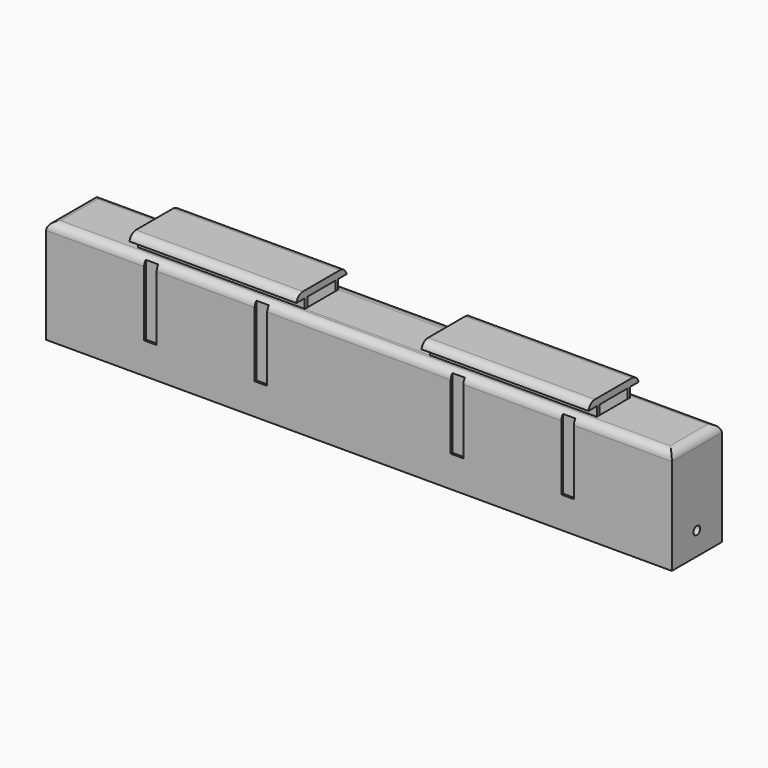
from build123d import *

# Parameters (mm, degrees)
F0_W           = 10.16
F0_H           = 2.54
F1_DEPTH       = 6.35
F2_DEPTH       = 0.635
F4_DEPTH       = 27.94
F6_R           = 0.254
F7_DEPTH       = 38.101
F8_T1_DEPTH    = 6.354829213
F8_T3_DEPTH    = 13.720829213
F10_DEPTH      = 9.652
F11_DEPTH      = 17.272
F12_W          = 2.5144716492
F12_H          = 3.5254987888
F13_DEPTH      = 3.81
F14_DEPTH      = 3.302
F16_DEPTH      = 10.16
F18_DEPTH      = 10.16
F20_DEPTH      = 10.16
F21_T1_DEPTH   = 12.6606557729
F23_DEPTH      = 10.16
F24_T1_DEPTH   = 12.6606557729
F24_2_T1_DEPTH = 8.0250460087
F24_2_T3_DEPTH = 8.0034146065
F24_2_T5_DEPTH = 8.0034146065
F24_2_T7_DEPTH = 8.0250460087
F25_W          = 7.62
F25_H          = 2.54
F26_DEPTH      = 4.5568268582
F27_W          = 7.62
F27_H          = 2.54
F28_DEPTH      = 4.5568268582
F0_W_2         = 0.762
F0_H_2         = 0.127
F29_DEPTH      = 1.905


# Not quite as in the source:
# - a fillet or chamfer that OpenCascade refuses, or shapes differently, is made with other operations: its cross-section is extruded or revolved along the edge and cut away or added


with BuildPart() as f1:
    # F0 (on Top) → F1 (new body)
    with BuildSketch(Plane.XY):
        Polygon((13.081, -1.905), (19.05, -1.905), (19.05, 1.905), (13.081, 1.905), (13.081, 1.778), (12.319, 1.778), (12.319, 1.905), (6.35, 1.905), (6.35, 1.778), (5.588, 1.778), (5.588, 1.905), (-5.588, 1.905), (-5.588, 1.778), (-6.35, 1.778), (-6.35, 1.905), (-12.319, 1.905), (-12.319, 1.778), (-13.081, 1.778), (-13.081, 1.905), (-19.05, 1.905), (-19.05, -1.905), (-13.081, -1.905), (-13.081, -1.778), (-12.319, -1.778), (-12.319, -1.905), (-6.35, -1.905), (-6.35, -1.778), (-5.588, -1.778), (-5.588, -1.905), (5.588, -1.905), (5.588, -1.778), (6.35, -1.778), (6.35, -1.905), (12.319, -1.905), (12.319, -1.778), (13.081, -1.778), align=None)
        with Locations((-8.89, 0)):
            Rectangle(F0_W, F0_H, mode=Mode.SUBTRACT)
        with Locations((8.89, 0)):
            Rectangle(F0_W, F0_H, mode=Mode.SUBTRACT)
    extrude(amount=F1_DEPTH)

    # F0 (on Top) → F2 (join)
    with BuildSketch(Plane.XY):
        with Locations((-8.89, 0)):
            Rectangle(F0_W, F0_H)
        with Locations((8.89, 0)):
            Rectangle(F0_W, F0_H)
    extrude(amount=F2_DEPTH)

    # F3 (on face) → F4 (cut, through all)
    with BuildSketch(Plane.YZ.offset(-13.97)):
        Polygon((-0.4982374667, 0.381), (0.4982374667, 0.381), (0.4982374667, 0.889), (1.27, 1.397), (1.27, 5.461), (-1.27, 5.461), (-1.27, 1.397), (-0.4982374667, 0.889), align=None)
    extrude(amount=F4_DEPTH, mode=Mode.SUBTRACT)

    # F6 (on face) → F7 (cut, through all)
    with BuildSketch(Plane(origin=(-19.05, 0, 0), x_dir=(0, -1, 0), z_dir=(-1, 0, 0))):
        with Locations((0, 1.397)):
            Circle(F6_R)
    extrude(amount=-F7_DEPTH, mode=Mode.SUBTRACT)

    # F8: fillet of radius 0.508 on 4 edges, made by hand

    # F8_s2 → F8_t1 (cut)
    with BuildSketch(Plane.XZ.offset(-3.1774146065)):
        with BuildLine():
            ThreePointArc((-18.5410343146, 6.3504), (-18.9012102448, 6.2012102448), (-19.0504, 5.8410343146))
            Line((-19.0504, 5.8410343146), (-19.1013365685, 5.8410343146))
            ThreePointArc((-19.1013365685, 5.8410343146), (-19.1009365685, 6.0955171573), (-19.1009365685, 6.35))
            Line((-19.1009365685, 6.35), (-19.05, 6.4009365685))
            ThreePointArc((-19.05, 6.4009365685), (-18.7955171573, 6.4009365685), (-18.5410343146, 6.4013365685))
            Line((-18.5410343146, 6.4013365685), (-18.5410343146, 6.3504))
        make_face()
        with BuildLine():
            ThreePointArc((19.0504, 5.8410343146), (18.9012102448, 6.2012102448), (18.5410343146, 6.3504))
            Line((18.5410343146, 6.3504), (18.5410343146, 6.4013365685))
            ThreePointArc((18.5410343146, 6.4013365685), (18.7955171573, 6.4009365685), (19.05, 6.4009365685))
            Line((19.05, 6.4009365685), (19.1009365685, 6.35))
            ThreePointArc((19.1009365685, 6.35), (19.1009365685, 6.0955171573), (19.1013365685, 5.8410343146))
            Line((19.1013365685, 5.8410343146), (19.0504, 5.8410343146))
        make_face()
    extrude(amount=F8_T1_DEPTH, mode=Mode.SUBTRACT)

    # F8_s4 → F8_t3 (cut)
    with BuildSketch(Plane.YZ.offset(-6.8604146065)):
        with BuildLine():
            ThreePointArc((1.3960343146, 6.3504), (1.7562102448, 6.2012102448), (1.9054, 5.8410343146))
            Line((1.9054, 5.8410343146), (1.9563365685, 5.8410343146))
            ThreePointArc((1.9563365685, 5.8410343146), (1.9559365685, 6.0955171573), (1.9559365685, 6.35))
            Line((1.9559365685, 6.35), (1.905, 6.4009365685))
            ThreePointArc((1.905, 6.4009365685), (1.6505171573, 6.4009365685), (1.3960343146, 6.4013365685))
            Line((1.3960343146, 6.4013365685), (1.3960343146, 6.3504))
        make_face()
        with BuildLine():
            ThreePointArc((-1.3960343146, 6.3504), (-1.7562102448, 6.2012102448), (-1.9054, 5.8410343146))
            Line((-1.9054, 5.8410343146), (-1.9563365685, 5.8410343146))
            ThreePointArc((-1.9563365685, 5.8410343146), (-1.9559365685, 6.0955171573), (-1.9559365685, 6.35))
            Line((-1.9559365685, 6.35), (-1.905, 6.4009365685))
            ThreePointArc((-1.905, 6.4009365685), (-1.6505171573, 6.4009365685), (-1.3960343146, 6.4013365685))
            Line((-1.3960343146, 6.4013365685), (-1.3960343146, 6.3504))
        make_face()
    extrude(amount=F8_T3_DEPTH, mode=Mode.SUBTRACT)


with BuildPart() as f10:
    # F9 (on face) → F10 (new body, through all)
    with BuildSketch(Plane(origin=(-3.81, 0, 0), x_dir=(0, -1, 0), z_dir=(-1, 0, 0))):
        with BuildLine():
            Line((-0.0880359173, 1.4812426976), (-0.381, 5.207))
            ThreePointArc((-0.381, 5.207), (-0.9198153673, 4.9838153673), (-1.143, 4.445))
            Line((-1.143, 4.445), (-1.143, 1.397))
            Line((-1.143, 1.397), (-0.4176268994, 0.8964751032))
            ThreePointArc((-0.4176268994, 0.8964751032), (0, 0.4231398893), (0.4176268994, 0.8964751032))
            Line((0.4176268994, 0.8964751032), (1.143, 1.397))
            Line((1.143, 1.397), (1.143, 4.445))
            ThreePointArc((1.143, 4.445), (0.9198153673, 4.9838153673), (0.381, 5.207))
            Line((0.381, 5.207), (0.0880359173, 1.4812426976))
            ThreePointArc((0.0880359173, 1.4812426976), (0.1267060772, 1.4088201678), (0.0771916931, 1.3433317729))
            Line((0.0771916931, 1.3433317729), (0.0768500527, 1.338986977))
            Line((0.0768500527, 1.338986977), (0.0526172437, 1.0308073381))
            ThreePointArc((0.0526172437, 1.0308073381), (0, 0.6500122176), (-0.0526172437, 1.0308073381))
            Line((-0.0526172437, 1.0308073381), (-0.0768500527, 1.338986977))
            Line((-0.0768500527, 1.338986977), (-0.0771916931, 1.3433317729))
            ThreePointArc((-0.0771916931, 1.3433317729), (-0.1904525618, 1.4038076485), (-0.0880359173, 1.4812426976))
        make_face()
    extrude(amount=F10_DEPTH)

    # F11 (add, through all): a face of the model
    f11_faces = [f10.faces().sort_by_distance(p)[0] for p in [
        (-3.81, 0, 0.5969923029),
    ]]
    extrude(f11_faces, amount=F11_DEPTH)

    # F12 (on Right) → F13 (cut, symmetric)
    with BuildSketch(Plane.YZ):
        with Locations((-0.0007677008, 3.5559225362)):
            Rectangle(F12_W, F12_H)
    extrude(amount=F13_DEPTH, both=True, mode=Mode.SUBTRACT)


with BuildPart() as f14:
    # F14 (new): a face of the model
    f14_faces = [f1.part.faces().sort_by_distance(p)[0] for p in [
        (0, 0, 5.461),
    ]]
    extrude(f14_faces, amount=F14_DEPTH)

    # F27 (on face) → F28 (join, through all)
    with BuildSketch(Plane.XY.offset(1.7931731418)):
        Rectangle(F27_W, F27_H)
    extrude(amount=F28_DEPTH)


with BuildPart() as f1_1:
    add(f1.part)

    # F15 (on face) → F16 (cut, through all)
    with BuildSketch(Plane.YZ.offset(-13.97)):
        with BuildLine():
            Line((1.27, 4.572), (1.27, 4.318))
            ThreePointArc((1.27, 4.318), (1.397, 4.445), (1.27, 4.572))
        make_face()
        with BuildLine():
            ThreePointArc((-1.27, 4.572), (-1.397, 4.445), (-1.27, 4.318))
            Line((-1.27, 4.318), (-1.27, 4.572))
        make_face()
        with BuildLine():
            Line((-1.27, 4.953), (-1.27, 5.207))
            ThreePointArc((-1.27, 5.207), (-1.397, 5.08), (-1.27, 4.953))
        make_face()
        with BuildLine():
            ThreePointArc((1.27, 4.953), (1.397, 5.08), (1.27, 5.207))
            Line((1.27, 5.207), (1.27, 4.953))
        make_face()
    extrude(amount=F16_DEPTH, mode=Mode.SUBTRACT)

    # F17 (on face) → F18 (cut, through all)
    with BuildSketch(Plane(origin=(13.97, 0, 0), x_dir=(0, -1, 0), z_dir=(-1, 0, 0))):
        with BuildLine():
            Line((1.27, 4.5734065802), (1.27, 4.3194065802))
            ThreePointArc((1.27, 4.3194065802), (1.397, 4.4464065802), (1.27, 4.5734065802))
        make_face()
        with BuildLine():
            ThreePointArc((-1.27, 4.5734065802), (-1.397, 4.4464065802), (-1.27, 4.3194065802))
            Line((-1.27, 4.3194065802), (-1.27, 4.5734065802))
        make_face()
        with BuildLine():
            Line((-1.27, 4.9544065802), (-1.27, 5.2084065802))
            ThreePointArc((-1.27, 5.2084065802), (-1.397, 5.0814065802), (-1.27, 4.9544065802))
        make_face()
        with BuildLine():
            ThreePointArc((1.27, 4.9544065802), (1.397, 5.0814065802), (1.27, 5.2084065802))
            Line((1.27, 5.2084065802), (1.27, 4.9544065802))
        make_face()
    extrude(amount=F18_DEPTH, mode=Mode.SUBTRACT)

    # F24#2: fillet of radius 0.508 on 8 edges, made by hand

    # F24_2_s2 → F24_2_t1 (cut)
    with BuildSketch(Plane.YZ.offset(11.8085853935)):
        with BuildLine():
            ThreePointArc((-1.9054, 5.8410343146), (-1.7562102448, 6.2012102448), (-1.3960343146, 6.3504))
            Line((-1.3960343146, 6.3504), (-1.3960343146, 6.4013365685))
            ThreePointArc((-1.3960343146, 6.4013365685), (-1.6505171573, 6.4009365685), (-1.905, 6.4009365685))
            Line((-1.905, 6.4009365685), (-1.9559365685, 6.35))
            ThreePointArc((-1.9559365685, 6.35), (-1.9559365685, 6.0955171573), (-1.9563365685, 5.8410343146))
            Line((-1.9563365685, 5.8410343146), (-1.9054, 5.8410343146))
        make_face()
        with BuildLine():
            ThreePointArc((1.3960343146, 6.3504), (1.7562102448, 6.2012102448), (1.9054, 5.8410343146))
            Line((1.9054, 5.8410343146), (1.9563365685, 5.8410343146))
            ThreePointArc((1.9563365685, 5.8410343146), (1.9559365685, 6.0955171573), (1.9559365685, 6.35))
            Line((1.9559365685, 6.35), (1.905, 6.4009365685))
            ThreePointArc((1.905, 6.4009365685), (1.6505171573, 6.4009365685), (1.3960343146, 6.4013365685))
            Line((1.3960343146, 6.4013365685), (1.3960343146, 6.3504))
        make_face()
    extrude(amount=F24_2_T1_DEPTH, mode=Mode.SUBTRACT)

    # F24_2_s4 → F24_2_t3 (cut)
    with BuildSketch(Plane.YZ.offset(5.588)):
        with BuildLine():
            ThreePointArc((-1.3960343146, 6.3504), (-1.7562102448, 6.2012102448), (-1.9054, 5.8410343146))
            Line((-1.9054, 5.8410343146), (-1.9563365685, 5.8410343146))
            ThreePointArc((-1.9563365685, 5.8410343146), (-1.9559365685, 6.0955171573), (-1.9559365685, 6.35))
            Line((-1.9559365685, 6.35), (-1.905, 6.4009365685))
            ThreePointArc((-1.905, 6.4009365685), (-1.6505171573, 6.4009365685), (-1.3960343146, 6.4013365685))
            Line((-1.3960343146, 6.4013365685), (-1.3960343146, 6.3504))
        make_face()
        with BuildLine():
            ThreePointArc((1.3960343146, 6.3504), (1.7562102448, 6.2012102448), (1.9054, 5.8410343146))
            Line((1.9054, 5.8410343146), (1.9563365685, 5.8410343146))
            ThreePointArc((1.9563365685, 5.8410343146), (1.9559365685, 6.0955171573), (1.9559365685, 6.35))
            Line((1.9559365685, 6.35), (1.905, 6.4009365685))
            ThreePointArc((1.905, 6.4009365685), (1.6505171573, 6.4009365685), (1.3960343146, 6.4013365685))
            Line((1.3960343146, 6.4013365685), (1.3960343146, 6.3504))
        make_face()
    extrude(amount=F24_2_T3_DEPTH, mode=Mode.SUBTRACT)

    # F24_2_s6 → F24_2_t5 (cut)
    with BuildSketch(Plane.YZ.offset(-13.5914146065)):
        with BuildLine():
            ThreePointArc((-1.3960343146, 6.3504), (-1.7562102448, 6.2012102448), (-1.9054, 5.8410343146))
            Line((-1.9054, 5.8410343146), (-1.9563365685, 5.8410343146))
            ThreePointArc((-1.9563365685, 5.8410343146), (-1.9559365685, 6.0955171573), (-1.9559365685, 6.35))
            Line((-1.9559365685, 6.35), (-1.905, 6.4009365685))
            ThreePointArc((-1.905, 6.4009365685), (-1.6505171573, 6.4009365685), (-1.3960343146, 6.4013365685))
            Line((-1.3960343146, 6.4013365685), (-1.3960343146, 6.3504))
        make_face()
        with BuildLine():
            ThreePointArc((1.3960343146, 6.3504), (1.7562102448, 6.2012102448), (1.9054, 5.8410343146))
            Line((1.9054, 5.8410343146), (1.9563365685, 5.8410343146))
            ThreePointArc((1.9563365685, 5.8410343146), (1.9559365685, 6.0955171573), (1.9559365685, 6.35))
            Line((1.9559365685, 6.35), (1.905, 6.4009365685))
            ThreePointArc((1.905, 6.4009365685), (1.6505171573, 6.4009365685), (1.3960343146, 6.4013365685))
            Line((1.3960343146, 6.4013365685), (1.3960343146, 6.3504))
        make_face()
    extrude(amount=F24_2_T5_DEPTH, mode=Mode.SUBTRACT)

    # F24_2_s8 → F24_2_t7 (cut)
    with BuildSketch(Plane.YZ.offset(-19.8336314022)):
        with BuildLine():
            ThreePointArc((-1.3960343146, 6.3504), (-1.7562102448, 6.2012102448), (-1.9054, 5.8410343146))
            Line((-1.9054, 5.8410343146), (-1.9563365685, 5.8410343146))
            ThreePointArc((-1.9563365685, 5.8410343146), (-1.9559365685, 6.0955171573), (-1.9559365685, 6.35))
            Line((-1.9559365685, 6.35), (-1.905, 6.4009365685))
            ThreePointArc((-1.905, 6.4009365685), (-1.6505171573, 6.4009365685), (-1.3960343146, 6.4013365685))
            Line((-1.3960343146, 6.4013365685), (-1.3960343146, 6.3504))
        make_face()
        with BuildLine():
            ThreePointArc((1.3960343146, 6.3504), (1.7562102448, 6.2012102448), (1.9054, 5.8410343146))
            Line((1.9054, 5.8410343146), (1.9563365685, 5.8410343146))
            ThreePointArc((1.9563365685, 5.8410343146), (1.9559365685, 6.0955171573), (1.9559365685, 6.35))
            Line((1.9559365685, 6.35), (1.905, 6.4009365685))
            ThreePointArc((1.905, 6.4009365685), (1.6505171573, 6.4009365685), (1.3960343146, 6.4013365685))
            Line((1.3960343146, 6.4013365685), (1.3960343146, 6.3504))
        make_face()
    extrude(amount=F24_2_T7_DEPTH, mode=Mode.SUBTRACT)

    # F25 (on face) → F26 (cut, through all)
    with BuildSketch(Plane.XY.offset(6.35)):
        Rectangle(F25_W, F25_H)
    extrude(amount=-F26_DEPTH, mode=Mode.SUBTRACT)

    # F0 (on Top) → F29 (join)
    with BuildSketch(Plane.XY):
        with Locations((-12.7, -1.8415)):
            Rectangle(F0_W_2, F0_H_2)
        with Locations((-5.969, -1.8415)):
            Rectangle(F0_W_2, F0_H_2)
        with Locations((-5.969, 1.8415)):
            Rectangle(F0_W_2, F0_H_2)
        with Locations((-12.7, 1.8415)):
            Rectangle(F0_W_2, F0_H_2)
        with Locations((5.969, -1.8415)):
            Rectangle(F0_W_2, F0_H_2)
        with Locations((12.7, -1.8415)):
            Rectangle(F0_W_2, F0_H_2)
        with Locations((12.7, 1.8415)):
            Rectangle(F0_W_2, F0_H_2)
        with Locations((5.969, 1.8415)):
            Rectangle(F0_W_2, F0_H_2)
    extrude(amount=F29_DEPTH)


with BuildPart() as f20:
    # F19 (on face) → F20 (new body, through all)
    with BuildSketch(Plane(origin=(13.97, 0, 0), x_dir=(0, -1, 0), z_dir=(-1, 0, 0))):
        with BuildLine():
            Line((-1.27, 4.9036065802), (-1.27, 3.7397078704))
            Line((-1.27, 3.7397078704), (-1.0667999741, 3.7397078704))
            Line((-1.0667999741, 3.7397078704), (-1.0667999741, 3.9429078963))
            Line((-1.0667999741, 3.9429078963), (-1.0667999741, 6.9219944999))
            Line((-1.0667999741, 6.9219944999), (1.0667999741, 6.9219944999))
            Line((1.0667999741, 6.9219944999), (1.0667999741, 4.4092186605))
            Line((1.0667999741, 4.4092186605), (1.0667999741, 3.7397078704))
            Line((1.0667999741, 3.7397078704), (1.27, 3.7397078704))
            Line((1.27, 3.7397078704), (1.27, 4.9036065802))
            ThreePointArc((1.27, 4.9036065802), (1.397, 5.0306065802), (1.27, 5.1576065802))
            Line((1.27, 5.1576065802), (1.27, 5.5386065802))
            ThreePointArc((1.27, 5.5386065802), (1.397, 5.6656065802), (1.27, 5.7926065802))
            Line((1.27, 5.7926065802), (1.27, 6.9219944999))
            Line((1.27, 6.9219944999), (1.905, 6.9219944999))
            Line((1.905, 6.9219944999), (1.905, 7.340928074))
            Line((1.905, 7.340928074), (-1.905, 7.340928074))
            Line((-1.905, 7.340928074), (-1.905, 6.9219944999))
            Line((-1.905, 6.9219944999), (-1.27, 6.9219944999))
            Line((-1.27, 6.9219944999), (-1.27, 5.7926065802))
            ThreePointArc((-1.27, 5.7926065802), (-1.397, 5.6656065802), (-1.27, 5.5386065802))
            Line((-1.27, 5.5386065802), (-1.27, 5.1576065802))
            ThreePointArc((-1.27, 5.1576065802), (-1.397, 5.0306065802), (-1.27, 4.9036065802))
        make_face()
    extrude(amount=F20_DEPTH)

    # F21: fillet of radius 0.508 on 2 edges, made by hand

    # F21_s2 → F21_t1 (cut)
    with BuildSketch(Plane.YZ.offset(2.5596721136)):
        with BuildLine():
            ThreePointArc((1.905, 6.9219944999), (1.7310729653, 7.2223569791), (1.4048688454, 7.340928074))
            Line((1.4048688454, 7.340928074), (1.905, 7.340928074))
            Line((1.905, 7.340928074), (1.905, 6.9219944999))
        make_face()
        with BuildLine():
            ThreePointArc((-1.4048688454, 7.340928074), (-1.7310729653, 7.2223569791), (-1.905, 6.9219944999))
            Line((-1.905, 6.9219944999), (-1.905, 7.340928074))
            Line((-1.905, 7.340928074), (-1.4048688454, 7.340928074))
        make_face()
    extrude(amount=F21_T1_DEPTH, mode=Mode.SUBTRACT)


with BuildPart() as f23:
    # F22 (on face) → F23 (new body, through all)
    with BuildSketch(Plane.YZ.offset(-13.97)):
        with BuildLine():
            Line((-1.27, 4.9036112368), (-1.27, 3.739712527))
            Line((-1.27, 3.739712527), (-1.0667999741, 3.739712527))
            Line((-1.0667999741, 3.739712527), (-1.0667999741, 3.942912553))
            Line((-1.0667999741, 3.942912553), (-1.0667999741, 6.9219991565))
            Line((-1.0667999741, 6.9219991565), (1.0667999741, 6.9219991565))
            Line((1.0667999741, 6.9219991565), (1.0667999741, 4.4092233171))
            Line((1.0667999741, 4.4092233171), (1.0667999741, 3.739712527))
            Line((1.0667999741, 3.739712527), (1.27, 3.739712527))
            Line((1.27, 3.739712527), (1.27, 4.9036112368))
            ThreePointArc((1.27, 4.9036112368), (1.397, 5.0306112368), (1.27, 5.1576112368))
            Line((1.27, 5.1576112368), (1.27, 5.5386112368))
            ThreePointArc((1.27, 5.5386112368), (1.397, 5.6656112368), (1.27, 5.7926112368))
            Line((1.27, 5.7926112368), (1.27, 6.9219991565))
            Line((1.27, 6.9219991565), (1.905, 6.9219991565))
            Line((1.905, 6.9219991565), (1.905, 7.3409327306))
            Line((1.905, 7.3409327306), (-1.905, 7.3409327306))
            Line((-1.905, 7.3409327306), (-1.905, 6.9219991565))
            Line((-1.905, 6.9219991565), (-1.27, 6.9219991565))
            Line((-1.27, 6.9219991565), (-1.27, 5.7926112368))
            ThreePointArc((-1.27, 5.7926112368), (-1.397, 5.6656112368), (-1.27, 5.5386112368))
            Line((-1.27, 5.5386112368), (-1.27, 5.1576112368))
            ThreePointArc((-1.27, 5.1576112368), (-1.397, 5.0306112368), (-1.27, 4.9036112368))
        make_face()
    extrude(amount=F23_DEPTH)

    # F24: fillet of radius 0.508 on 2 edges, made by hand

    # F24_s2 → F24_t1 (cut)
    with BuildSketch(Plane.YZ.offset(-15.2203278864)):
        with BuildLine():
            ThreePointArc((-1.905, 6.9219991565), (-1.7310729653, 7.2223616357), (-1.4048688454, 7.3409327306))
            Line((-1.4048688454, 7.3409327306), (-1.905, 7.3409327306))
            Line((-1.905, 7.3409327306), (-1.905, 6.9219991565))
        make_face()
        with BuildLine():
            ThreePointArc((1.4048688454, 7.3409327306), (1.7310729653, 7.2223616357), (1.905, 6.9219991565))
            Line((1.905, 6.9219991565), (1.905, 7.3409327306))
            Line((1.905, 7.3409327306), (1.4048688454, 7.3409327306))
        make_face()
    extrude(amount=F24_T1_DEPTH, mode=Mode.SUBTRACT)


solid = Compound([f10.part, f14.part, f1_1.part, f20.part, f23.part])
